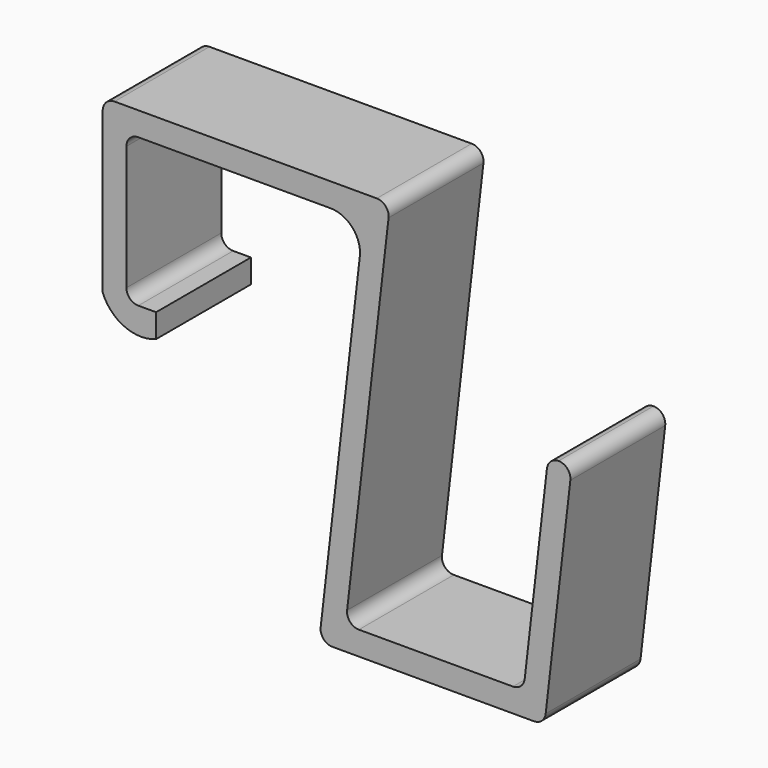
from build123d import *

# Parameters (mm, degrees)
F1_DEPTH    = 20
F2_R        = 2
F3_T1_DEPTH = 30
F3_T3_DEPTH = 31.2212666506
F3_T5_DEPTH = 28.9116499156
F4_R        = 5


# Not quite as in the source:
# - a fillet or chamfer that OpenCascade refuses, or shapes differently, is made with other operations: its cross-section is extruded or revolved along the edge and cut away or added


with BuildPart() as f1:
    # F0 (on Front) → F1 (new body)
    with BuildSketch(Plane.XZ):
        Polygon((-24, 29), (-24, 0), (-20, 0), (-20, 25), (20, 25), (12.4937456114, -40), (50.4937456114, -40), (55.1129790813, 0), (51.1129790813, 0), (46.9556689583, -36), (16.9556689583, -36), (24.461923347, 29), align=None)
        with BuildLine():
            Line((-20, 0), (-24, 0))
            ThreePointArc((-24, 0), (-20.3284271247, -3.8639610307), (-15, -4))
            Line((-15, -4), (-15, 0))
            Line((-15, 0), (-20, 0))
        make_face()
    extrude(amount=F1_DEPTH)

    # F2
    f2_edges = [f1.edges().sort_by_distance(p)[0] for p in [
        (-20, -10, 0),
        (-20, -10, 25),
        (16.955669, -10, -36),
        (46.955669, -10, -36),
    ]]
    fillet(f2_edges, radius=F2_R)

    # F3: fillet of radius 2 on 6 edges, made by hand

    # F3_s2 → F3_t1 (cut)
    with BuildSketch(Plane.XZ.offset(-5)):
        with BuildLine():
            ThreePointArc((-22, 29), (-23.4142135624, 28.4142135624), (-24, 27))
            Line((-24, 27), (-24, 29))
            Line((-24, 29), (-22, 29))
        make_face()
    extrude(amount=F3_T1_DEPTH, mode=Mode.SUBTRACT)

    # F3_s4 → F3_t3 (cut)
    with BuildSketch(Plane.XZ.offset(-5.6106333253)):
        with BuildLine():
            ThreePointArc((24.2044661111, 26.7705631246), (23.7107999092, 28.3306250879), (22.2176700169, 29))
            Line((22.2176700169, 29), (24.461923347, 29))
            Line((24.461923347, 29), (24.2044661111, 26.7705631246))
        make_face()
        with BuildLine():
            ThreePointArc((14.7379989415, -40), (13.2448690491, -39.3306250879), (12.7512028472, -37.7705631246))
            Line((12.7512028472, -37.7705631246), (12.4937456114, -40))
            Line((12.4937456114, -40), (14.7379989415, -40))
        make_face()
        with BuildLine():
            ThreePointArc((52.8687257512, 0), (54.3618556435, -0.6693749121), (54.8555218454, -2.2294368754))
            Line((54.8555218454, -2.2294368754), (55.1129790813, 0))
            Line((55.1129790813, 0), (52.8687257512, 0))
        make_face()
    extrude(amount=F3_T3_DEPTH, mode=Mode.SUBTRACT)

    # F3_s6 → F3_t5 (cut)
    with BuildSketch(Plane.XZ.offset(-4.4558249578)):
        with BuildLine():
            ThreePointArc((50.6982117225, -38.2294368754), (50.0420407161, -39.4931298923), (48.7114156282, -40))
            Line((48.7114156282, -40), (50.4937456114, -40))
            Line((50.4937456114, -40), (50.6982117225, -38.2294368754))
        make_face()
        with BuildLine():
            ThreePointArc((50.9085129701, -1.7705631246), (51.5646839765, -0.5068701077), (52.8953090644, 0))
            Line((52.8953090644, 0), (51.1129790813, 0))
            Line((51.1129790813, 0), (50.9085129701, -1.7705631246))
        make_face()
    extrude(amount=F3_T5_DEPTH, mode=Mode.SUBTRACT)

    # F4
    f4_edges = [f1.edges().sort_by_distance(p)[0] for p in [
        (20, -10, 25),
    ]]
    fillet(f4_edges, radius=F4_R)


solid = f1.part
